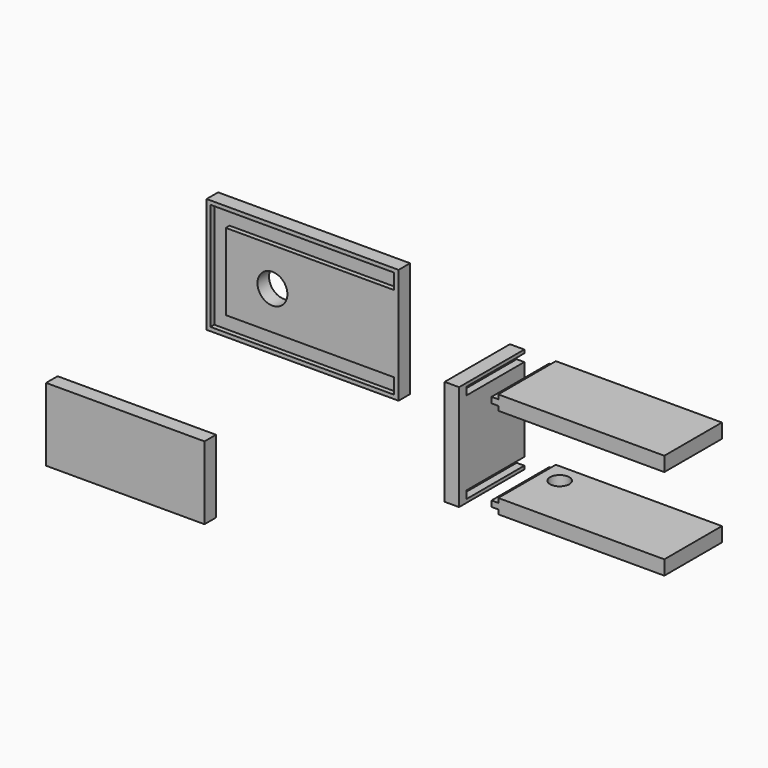
from build123d import *

# Parameters (mm, degrees)
F0_R     = 19.7613438491
F0_W     = 222.25
F0_H     = 20.32
F0_W_2   = 6.35
F1_DEPTH = 19.05
F2_W     = 222.25
F2_H     = 20.32
F3_DEPTH = 6.35
F4_DEPTH = 95.25
F0_W_3   = 8.89
F0_H_2   = 7.62
F5_R     = 12.7
F6_DEPTH = 191.0149866296
F7_W     = 19.05
F7_H     = 139.7
F8_DEPTH = 12.7
F0_W_4   = 209.55
F0_H_3   = 96.52
F9_DEPTH = 19.05


# Not quite as in the source:
# - a feature names something its author has since deleted; it is built from what else it names


with BuildPart() as f1:
    # F0 (on Front) → F1 (new body)
    with BuildSketch(Plane.XZ):
        Polygon((167.8302989408, 95.9372372214), (167.8302989408, 116.2572372214), (-74.7397010592, 116.2572372214), (-74.7397010592, -25.9827627786), (-54.4197010592, -25.9827627786), (-54.4197010592, -5.6627627786), (-54.4197010592, 95.9372372214), align=None)
        Polygon((174.1802989408, -5.6627627786), (174.1802989408, 95.9372372214), (167.8302989408, 95.9372372214), (-54.4197010592, 95.9372372214), (-54.4197010592, -5.6627627786), (167.8302989408, -5.6627627786), align=None)
        with Locations((7.3118018918, 45.1372372214)):
            Circle(F0_R, mode=Mode.SUBTRACT)
        with Locations((56.7052989408, -15.8227627786)):
            Rectangle(F0_W, F0_H)
        Polygon((174.1802989408, 121.3372372214), (-79.8197010592, 121.3372372214), (-79.8197010592, -31.0627627786), (174.1802989408, -31.0627627786), (174.1802989408, -25.9827627786), (167.8302989408, -25.9827627786), (-54.4197010592, -25.9827627786), (-74.7397010592, -25.9827627786), (-74.7397010592, 116.2572372214), (167.8302989408, 116.2572372214), (174.1802989408, 116.2572372214), align=None)
        with Locations((171.0052989408, 106.0972372214)):
            Rectangle(F0_W_2, F0_H)
        with Locations((171.0052989408, -15.8227627786)):
            Rectangle(F0_W_2, F0_H)
    extrude(amount=F1_DEPTH)

    # F2 (on face) → F3 (cut)
    with BuildSketch(Plane.XZ.offset(19.05)):
        Polygon((-54.4197010592, 116.2572372214), (-74.7397010592, 116.2572372214), (-74.7397010592, -25.9827627786), (-54.4197010592, -25.9827627786), (-54.4197010592, -5.6627627786), (-54.4197010592, 95.9372372214), align=None)
        with Locations((56.7052989408, 106.0972372214)):
            Rectangle(F2_W, F2_H)
        with Locations((56.7052989408, -15.8227627786)):
            Rectangle(F2_W, F2_H)
    extrude(amount=-F3_DEPTH, mode=Mode.SUBTRACT)


with BuildPart() as f4:
    # F0 (on Front) → F4 (new body)
    with BuildSketch(Plane.XZ):
        Polygon((325.3248014927, 70.0232505918), (306.2748014927, 70.0232505918), (306.2748014927, -69.6767494082), (325.3248014927, -69.6767494082), (325.3248014927, -65.2317494082), (315.1758867264, -65.2317494082), (315.1758867264, -55.0717494082), (325.3248014927, -55.0717494082), (325.3248014927, 55.4182505918), (315.1758867264, 55.4182505918), (315.1758867264, 65.5782505918), (325.3248014927, 65.5782505918), align=None)
    extrude(amount=F4_DEPTH)

    # F7 (on face) → F8 (join)
    with BuildSketch(Plane.XZ.offset(95.25)):
        with Locations((315.7998014927, 0.1732505918)):
            Rectangle(F7_W, F7_H)
    extrude(amount=F8_DEPTH)


with BuildPart() as f4b:
    # F0 (on Front) → F4, piece 2 (new body)
    with BuildSketch(Plane.XZ):
        Polygon((586.7272095299, 70.0232505918), (367.0172095299, 70.0232505918), (367.0172095299, 64.3082505918), (367.0172095299, 56.6882505918), (367.0172095299, 50.9732505918), (586.7272095299, 50.9732505918), align=None)
        with Locations((362.5722095299, 60.4982505918)):
            Rectangle(F0_W_3, F0_H_2)
    extrude(amount=F4_DEPTH)


with BuildPart() as f4c:
    # F0 (on Front) → F4, piece 3 (new body)
    with BuildSketch(Plane.XZ):
        Polygon((586.7272095299, -50.6267494082), (367.0172095299, -50.6267494082), (367.0172095299, -56.3417494082), (367.0172095299, -63.9617494082), (367.0172095299, -69.6767494082), (586.7272095299, -69.6767494082), align=None)
        with Locations((362.5722095299, -60.1517494082)):
            Rectangle(F0_W_3, F0_H_2)
    extrude(amount=F4_DEPTH)

    # F5 (on face) → F6 (cut, through all)
    with BuildSketch(Plane(origin=(0, 0, -69.6767494082), x_dir=(1, 0, 0), z_dir=(0, 0, -1))):
        with Locations((392.4172095299, 25.4)):
            Circle(F5_R)
    extrude(amount=-F6_DEPTH, mode=Mode.SUBTRACT)


with BuildPart() as f9:
    # F0 (on Front) → F9 (new body)
    with BuildSketch(Plane.XZ):
        with Locations((-187.3835738659, -210.1594242954)):
            Rectangle(F0_W_4, F0_H_3)
    extrude(amount=F9_DEPTH)


solid = Compound([f1.part, f4.part, f4b.part, f4c.part, f9.part])
